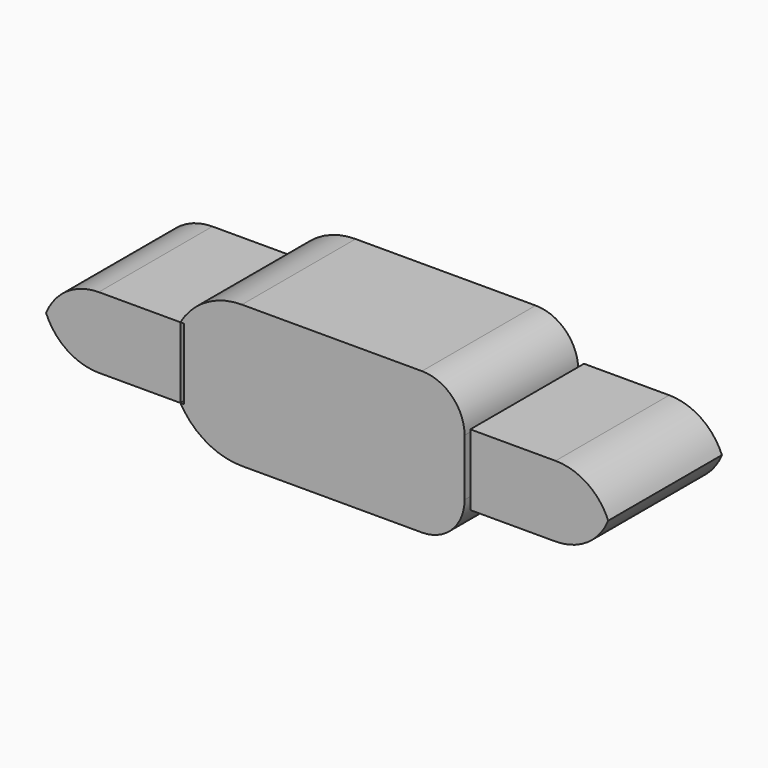
from build123d import *

# Parameters (mm, degrees)
F0_W          = 12.7
F0_H          = 6.35
F1_DEPTH      = 12.7
F0_W_2        = 12.37452721
F2_T1_DEPTH   = 40.1963065702
F3_T1_DEPTH   = 38.1
F3_2_T1_DEPTH = 38.1
F4_R          = 3.81


# Not quite as in the source:
# - a fillet or chamfer that OpenCascade refuses, or shapes differently, is made with other operations: its cross-section is extruded or revolved along the edge and cut away or added


with BuildPart() as f1:
    # F0 (on Front) → F1 (new body)
    with BuildSketch(Plane.XZ):
        with Locations((19.5622947067, 0)):
            Rectangle(F0_W, F0_H)
    extrude(amount=F1_DEPTH)

    # F3: fillet of radius 5.08 on 2 edges, made by hand

    # F3_s2 → F3_t1 (cut)
    with BuildSketch(Plane.XZ.offset(-12.7)):
        with BuildLine():
            ThreePointArc((20.8322947067, -3.175), (24.4243971551, -1.6871024484), (25.9122947067, 1.905))
            Line((25.9122947067, 1.905), (25.9122947067, -3.175))
            Line((25.9122947067, -3.175), (20.8322947067, -3.175))
        make_face()
        with BuildLine():
            ThreePointArc((25.9122947067, -1.905), (24.4243971551, 1.6871024484), (20.8322947067, 3.175))
            Line((20.8322947067, 3.175), (25.9122947067, 3.175))
            Line((25.9122947067, 3.175), (25.9122947067, -1.905))
        make_face()
    extrude(amount=F3_T1_DEPTH, mode=Mode.SUBTRACT)


with BuildPart() as f1b:
    # F0 (on Front) → F1, piece 2 (new body)
    with BuildSketch(Plane.XZ):
        with Locations((-18.887263605, 0)):
            Rectangle(F0_W_2, F0_H)
    extrude(amount=F1_DEPTH)

    # F3#2: fillet of radius 5.08 on 2 edges, made by hand

    # F3_2_s2 → F3_2_t1 (cut)
    with BuildSketch(Plane.XZ.offset(-12.7)):
        with BuildLine():
            ThreePointArc((-25.07452721, 1.905), (-23.5866296584, -1.6871024484), (-19.99452721, -3.175))
            Line((-19.99452721, -3.175), (-25.07452721, -3.175))
            Line((-25.07452721, -3.175), (-25.07452721, 1.905))
        make_face()
        with BuildLine():
            ThreePointArc((-19.99452721, 3.175), (-23.5866296584, 1.6871024484), (-25.07452721, -1.905))
            Line((-25.07452721, -1.905), (-25.07452721, 3.175))
            Line((-25.07452721, 3.175), (-19.99452721, 3.175))
        make_face()
    extrude(amount=F3_2_T1_DEPTH, mode=Mode.SUBTRACT)


with BuildPart() as f1c:
    # F0 (on Front) → F1, piece 3 (new body)
    with BuildSketch(Plane.XZ):
        Polygon((-12.7, -6.35), (12.7, -6.35), (12.7, 6.35), (-12.7, 6.35), (-12.7, 3.175), (-12.37452721, 3.175), (-12.37452721, -3.175), (-12.7, -3.175), align=None)
    extrude(amount=F1_DEPTH)

    # F2: fillet of radius 6.35 on 2 edges, made by hand

    # F2_s2 → F2_t1 (cut)
    with BuildSketch(Plane.XZ.offset(-13.7481532851)):
        with BuildLine():
            ThreePointArc((-7.200738686, 6.35), (-10.375738686, 5.499261314), (-12.7, 3.175))
            Line((-12.7, 3.175), (-12.7, 6.35))
            Line((-12.7, 6.35), (-7.200738686, 6.35))
        make_face()
        with BuildLine():
            ThreePointArc((-7.200738686, -6.35), (-10.375738686, -5.499261314), (-12.7, -3.175))
            Line((-12.7, -3.175), (-12.7, -6.35))
            Line((-12.7, -6.35), (-7.200738686, -6.35))
        make_face()
    extrude(amount=F2_T1_DEPTH, mode=Mode.SUBTRACT)

    # F4
    f4_edges = [f1c.edges().sort_by_distance(p)[0] for p in [
        (12.7, -6.35, 6.35),
        (12.7, -6.35, -6.35),
    ]]
    fillet(f4_edges, radius=F4_R)


solid = Compound([f1.part, f1b.part, f1c.part])
